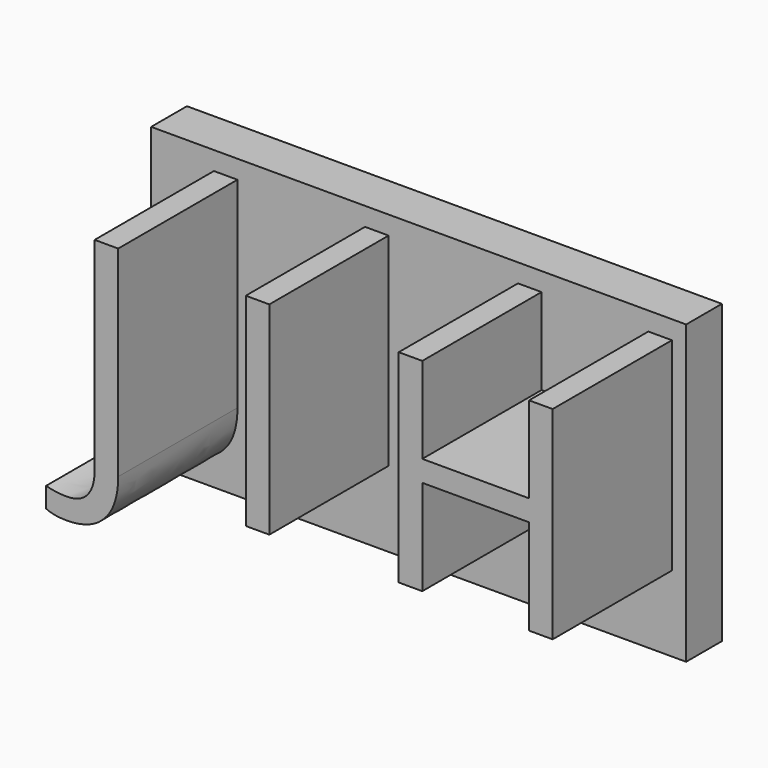
from build123d import *

# Parameters (mm, degrees)
F0_W         = 91.1634713411
F0_H         = 50.605405122
F1_DEPTH     = 7.62
F2_TEXT_SIZE = 48.3931456175
F3_DEPTH     = 25.4


# Not quite as in the source:
# - a feature names something its author has since deleted; it is built from what else it names
# - Text() gives the source's letters only with a copy of the font that has no kerning and outlines rounded to 1/6400 em; it was checked with that copy


with BuildPart() as f1:
    # F0 (on Front) → F1 (new body)
    with BuildSketch(Plane.XZ):
        with Locations((45.5817356706, 25.302702561)):
            Rectangle(F0_W, F0_H)
    extrude(amount=F1_DEPTH)

    # F2 (on face) → F3 (join)
    with BuildSketch(Plane.XZ.offset(7.62)):
        with Locations((6.1964557972, 12.9043650813)):
            Text('J I H', F2_TEXT_SIZE, font='Open Sans', text_align=(TextAlign.LEFT, TextAlign.BOTTOM))
    extrude(amount=F3_DEPTH)


solid = f1.part
